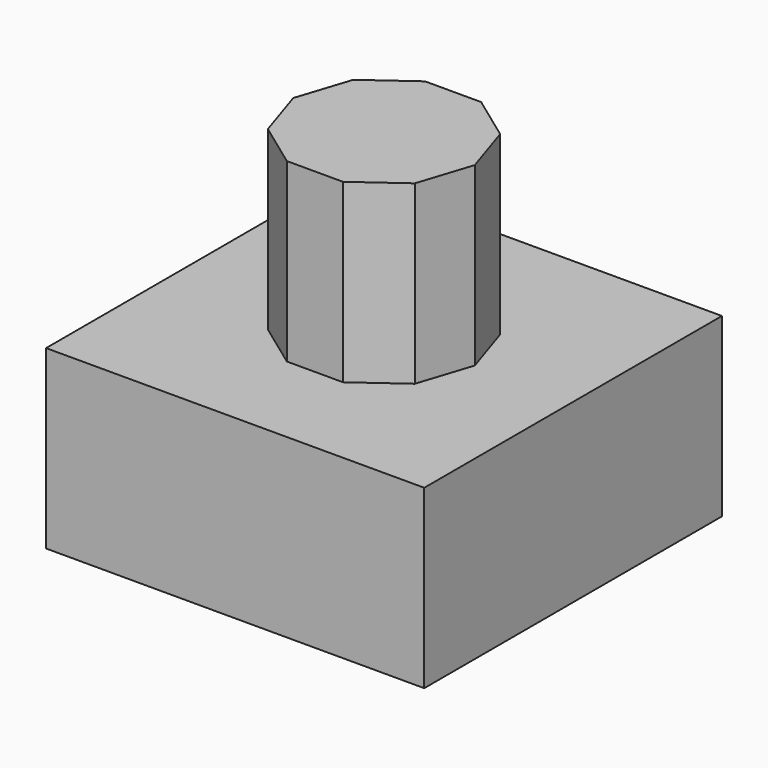
from build123d import *

# Parameters (mm, degrees)
F0_W     = 81.6473141313
F0_H     = 80.3374648094
F1_DEPTH = 38.1
F3_DEPTH = 76.2


# Not quite as in the source:
# - the program builds the solid bodies; features that only make, move or delete a surface that nothing else refers to are left out


with BuildPart() as f1:
    # F0 (on Top) → F1 (new body)
    with BuildSketch(Plane.XY):
        Rectangle(F0_W, F0_H)
        Polygon((-15.8581690014, 11.5216341958), (-6.0572815592, 18.6423957348), (6.0572815592, 18.6423957348), (15.8581690014, 11.5216341958), (19.6017748844, 0), (15.8581690014, -11.5216341958), (6.0572815592, -18.6423957348), (-6.0572815592, -18.6423957348), (-15.8581690014, -11.5216341958), (-19.6017748844, 0), align=None, mode=Mode.SUBTRACT)
    extrude(amount=F1_DEPTH)

    # F0 (on Top) → F3 (join)
    with BuildSketch(Plane.XY):
        Polygon((6.0572815592, 18.6423957348), (-6.0572815592, 18.6423957348), (-15.8581690014, 11.5216341958), (-19.6017748844, 0), (-15.8581690014, -11.5216341958), (-6.0572815592, -18.6423957348), (6.0572815592, -18.6423957348), (15.8581690014, -11.5216341958), (19.6017748844, 0), (15.8581690014, 11.5216341958), align=None)
    extrude(amount=F3_DEPTH)


solid = f1.part
